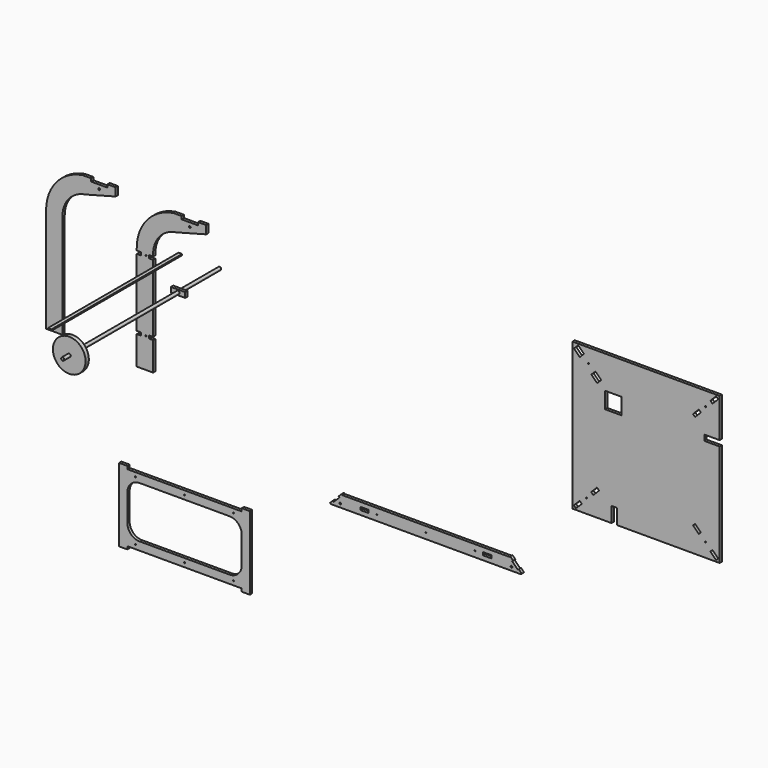
from build123d import *

# Parameters (mm, degrees)
F0_R          = 3.302
F0_R_2        = 5.588
F1_DEPTH      = 18.034
F0_W          = 50.8
F0_H          = 18.034
F0_W_2        = 101.6
F0_H_2        = 101.6
F0_W_3        = 88.9
F0_H_3        = 31.75
F0_R_3        = 9.525
F0_W_4        = 22.225
F0_H_4        = 7.62
F2_DEPTH      = 1016
F3_DEPTH      = 914.4
F3_DEPTH_BACK = 304.8
F5_START      = -50.8
F4_R          = 101.6
F4_R_2        = 9.525
F5_DEPTH      = 25.4


# Not quite as in the source:
# - a feature names something its author has since deleted; it is built from what else it names


with BuildPart() as f1:
    # F0 (on Front) → F1 (new body)
    with BuildSketch(Plane.XZ):
        with BuildLine():
            Line((-256.7524378796, -311.5848713337), (-256.7524378796, -489.3848713337))
            Line((-256.7524378796, -489.3848713337), (-155.1524378796, -489.3848713337))
            Line((-155.1524378796, -489.3848713337), (-155.1524378796, -311.5848713337))
            Line((-155.1524378796, -311.5848713337), (-180.5524378796, -311.5848713337))
            Line((-180.5524378796, -311.5848713337), (-180.5524378796, -293.5508713337))
            Line((-180.5524378796, -293.5508713337), (-155.1524378796, -293.5508713337))
            Line((-155.1524378796, -293.5508713337), (-155.1524378796, 127.5811286663))
            Line((-155.1524378796, 127.5811286663), (-180.5524378796, 127.5811286663))
            Line((-180.5524378796, 127.5811286663), (-180.5524378796, 145.6151286663))
            Line((-180.5524378796, 145.6151286663), (-155.1524378796, 145.6151286663))
            Line((-155.1524378796, 145.6151286663), (-155.1524378796, 159.8593657013))
            ThreePointArc((-155.1524378796, 159.8593657013), (-114.7622837077, 268.5646027694), (-13.1903100775, 324.5228666178))
            Line((-13.1903100775, 324.5228666178), (175.0475621204, 374.6868958044))
            Line((175.0475621204, 374.6868958044), (175.0475621204, 406.9811286663))
            Line((175.0475621204, 406.9811286663), (175.0475621204, 425.0151286663))
            Line((175.0475621204, 425.0151286663), (124.2475621204, 425.0151286663))
            Line((124.2475621204, 425.0151286663), (124.2475621204, 406.9811286663))
            Line((124.2475621204, 406.9811286663), (22.6475621204, 406.9811286663))
            Line((22.6475621204, 406.9811286663), (22.6475621204, 425.0151286663))
            Line((22.6475621204, 425.0151286663), (-28.1524378796, 425.0151286663))
            ThreePointArc((-28.1524378796, 425.0151286663), (-191.7126319353, 334.9061727512), (-256.7524378796, 159.8593657013))
            Line((-256.7524378796, 159.8593657013), (-256.7524378796, 145.6151286663))
            Line((-256.7524378796, 145.6151286663), (-231.3524378796, 145.6151286663))
            Line((-231.3524378796, 145.6151286663), (-231.3524378796, 127.5811286663))
            Line((-231.3524378796, 127.5811286663), (-256.7524378796, 127.5811286663))
            Line((-256.7524378796, 127.5811286663), (-256.7524378796, -293.5508713337))
            Line((-256.7524378796, -293.5508713337), (-231.3524378796, -293.5508713337))
            Line((-231.3524378796, -293.5508713337), (-231.3524378796, -311.5848713337))
            Line((-231.3524378796, -311.5848713337), (-256.7524378796, -311.5848713337))
        make_face()
        with Locations((-199.6024378796, -302.5678713337)):
            Circle(F0_R, mode=Mode.SUBTRACT)
        with Locations((-199.6024378796, 136.5981286663)):
            Circle(F0_R, mode=Mode.SUBTRACT)
        with Locations((73.4475621204, 381.5811286663)):
            Circle(F0_R_2, mode=Mode.SUBTRACT)
    extrude(amount=F1_DEPTH)


with BuildPart() as f1b:
    # F0 (on Front) → F1, piece 2 (new body)
    with BuildSketch(Plane.XZ):
        with BuildLine():
            ThreePointArc((-718.6880954381, 183.6058530265), (-678.2979412662, 292.3110900946), (-576.7259676359, 348.269353943))
            Line((-576.7259676359, 348.269353943), (-388.488095438, 398.4333831296))
            Line((-388.4880954381, 398.4333831296), (-388.4880954381, 430.7276159915))
            Line((-388.4880954381, 430.7276159915), (-388.4880954381, 448.7616159915))
            Line((-388.4880954381, 448.7616159915), (-439.2880954381, 448.7616159915))
            Line((-439.2880954381, 448.7616159915), (-439.2880954381, 430.7276159915))
            Line((-439.2880954381, 430.7276159915), (-540.8880954381, 430.7276159915))
            Line((-540.8880954381, 430.7276159915), (-540.8880954381, 448.7616159915))
            Line((-540.8880954381, 448.7616159915), (-591.6880954381, 448.7616159915))
            ThreePointArc((-591.6880954381, 448.7616159915), (-755.2482894938, 358.6526600765), (-820.2880954381, 183.6058530265))
            Line((-820.2880954381, 183.6058530265), (-820.2880954381, -465.6383840085))
            Line((-820.2880954381, -465.6383840085), (-718.6880954381, -465.6383840085))
            Line((-718.6880954381, -465.6383840085), (-718.6880954381, 183.6058530265))
        make_face()
        with Locations((-490.0880954381, 405.3276159915)):
            Circle(F0_R_2, mode=Mode.SUBTRACT)
    extrude(amount=F1_DEPTH)


with BuildPart() as f1c:
    # F0 (on Front) → F1, piece 3 (new body)
    with BuildSketch(Plane.XZ):
        Polygon((-315.3730721781, -1069.7679861069), (-366.1730721781, -1069.7679861069), (-366.1730721781, -1490.8999861069), (-315.3730721781, -1490.8999861069), (395.8269278219, -1490.8999861069), (446.6269278219, -1490.8999861069), (446.6269278219, -1069.7679861069), (395.8269278219, -1069.7679861069), align=None)
        with Locations((-264.5730721781, -1465.4999861069)):
            Circle(F0_R, mode=Mode.SUBTRACT)
        with Locations((40.2269278219, -1465.4999861069)):
            Circle(F0_R, mode=Mode.SUBTRACT)
        with BuildLine():
            ThreePointArc((-315.3730721781, -1196.7679861069), (-293.0546089045, -1142.8864493805), (-239.1730721781, -1120.5679861069))
            Line((-239.1730721781, -1120.5679861069), (319.6269278219, -1120.5679861069))
            ThreePointArc((319.6269278219, -1120.5679861069), (373.5084645483, -1142.8864493805), (395.8269278219, -1196.7679861069))
            Line((395.8269278219, -1196.7679861069), (395.8269278219, -1363.8999861069))
            ThreePointArc((395.8269278219, -1363.8999861069), (373.5084645483, -1417.7815228333), (319.6269278219, -1440.0999861069))
            Line((319.6269278219, -1440.0999861069), (-239.1730721781, -1440.0999861069))
            ThreePointArc((-239.1730721781, -1440.0999861069), (-293.0546089045, -1417.7815228333), (-315.3730721781, -1363.8999861069))
            Line((-315.3730721781, -1363.8999861069), (-315.3730721781, -1196.7679861069))
        make_face(mode=Mode.SUBTRACT)
        with Locations((-264.5730721781, -1095.1679861069)):
            Circle(F0_R, mode=Mode.SUBTRACT)
        with Locations((40.2269278219, -1095.1679861069)):
            Circle(F0_R, mode=Mode.SUBTRACT)
        with Locations((345.0269278219, -1465.4999861069)):
            Circle(F0_R, mode=Mode.SUBTRACT)
        with Locations((345.0269278219, -1095.1679861069)):
            Circle(F0_R, mode=Mode.SUBTRACT)
        with Locations((-340.7730721781, -1060.7509861069)):
            Rectangle(F0_W, F0_H)
        with Locations((421.2269278219, -1060.7509861069)):
            Rectangle(F0_W, F0_H)
        with Locations((421.2269278219, -1499.9169861069)):
            Rectangle(F0_W, F0_H)
        with Locations((-340.7730721781, -1499.9169861069)):
            Rectangle(F0_W, F0_H)
    extrude(amount=F1_DEPTH)


with BuildPart() as f1d:
    # F0 (on Front) → F1, piece 4 (new body)
    with BuildSketch(Plane.XZ):
        Polygon((2728.8376075736, -291.5323071868), (2728.8376075736, -385.9785684254), (3365.8825668832, -385.9785684254), (3365.8825668832, 251.3926928132), (3270.6325668832, 251.3926928132), (3270.6325668832, 286.3176928132), (3365.8825668832, 286.3176928132), (3365.8825668832, 528.4214315746), (2451.4825668832, 528.4214315746), (2451.4825668832, -385.9785684254), (2693.9126075736, -385.9785684254), (2693.9126075736, -291.5323071868), align=None)
        Polygon((2496.0684305155, -328.6407411012), (2508.8203942074, -341.3927047931), (2472.8993697231, -377.3137292774), (2460.1474060312, -364.5617655855), align=None, mode=Mode.SUBTRACT)
        with Locations((2538.3654368457, -299.0956984629)):
            Circle(F0_R, mode=Mode.SUBTRACT)
        Polygon((2603.8315039683, -220.8776676484), (2616.5834676602, -233.6296313403), (2580.662443176, -269.5506558246), (2567.910479484, -256.7986921326), align=None, mode=Mode.SUBTRACT)
        Polygon((3357.2177277351, -364.5617655855), (3344.4657640432, -377.3137292774), (3308.5447395589, -341.3927047931), (3321.2967032509, -328.6407411012), align=None, mode=Mode.SUBTRACT)
        Polygon((3249.4546542823, -256.7986921326), (3236.7026905904, -269.5506558246), (3200.7816661061, -233.6296313403), (3213.533629798, -220.8776676484), align=None, mode=Mode.SUBTRACT)
        with Locations((3278.9996969206, -299.0956984629)):
            Circle(F0_R, mode=Mode.SUBTRACT)
        with Locations((2705.4825668832, 274.4214315746)):
            Rectangle(F0_W_2, F0_H_2, mode=Mode.SUBTRACT)
        Polygon((2568.7111476991, 386.3110991977), (2594.2493832335, 411.7806722172), (2630.1704077178, 375.8596477329), (2604.6664803341, 350.3557203489), align=None, mode=Mode.SUBTRACT)
        with Locations((2551.796844501, 441.1701824532)):
            Circle(F0_R, mode=Mode.SUBTRACT)
        Polygon((2486.4863097807, 519.5437456699), (2522.407334265, 483.6227211856), (2496.9377612456, 458.0844856513), (2460.9823823967, 494.0398182862), align=None, mode=Mode.SUBTRACT)
        Polygon((3200.7816661061, 376.0724944895), (3236.7026905904, 411.9935189737), (3249.4546542823, 399.2415552818), (3213.533629798, 363.3205307975), align=None, mode=Mode.SUBTRACT)
        with Locations((3278.9996969206, 441.538561612)):
            Circle(F0_R, mode=Mode.SUBTRACT)
        Polygon((3321.2967032509, 471.0836042504), (3308.5447395589, 483.8355679423), (3344.4657640432, 519.7565924266), (3357.2177277351, 507.0046287346), align=None, mode=Mode.SUBTRACT)
    extrude(amount=F1_DEPTH)


with BuildPart() as f1e:
    # F0 (on Front) → F1, piece 5 (new body)
    with BuildSketch(Plane.XZ):
        Polygon((967.6722639506, -831.2486945482), (949.7117517085, -849.2092067904), (2130.8015917085, -849.2092067904), (2112.8410794663, -831.2486945482), (2076.9200549821, -795.3276700639), (2058.9595427399, -777.3671578218), (1021.553800677, -777.3671578218), (1003.5932884349, -795.3276700639), align=None)
        with Locations((1008.0834164954, -826.7585664877)):
            Circle(F0_R_2, mode=Mode.SUBTRACT)
        with Locations((1159.2566717085, -813.2881823061)):
            Rectangle(F0_W, F0_H, mode=Mode.SUBTRACT)
        with Locations((1235.4566717085, -813.2881823061)):
            Circle(F0_R, mode=Mode.SUBTRACT)
        with Locations((1540.2566717085, -813.2881823061)):
            Circle(F0_R, mode=Mode.SUBTRACT)
        with Locations((1845.0566717085, -813.2881823061)):
            Circle(F0_R, mode=Mode.SUBTRACT)
        with Locations((1921.2566717085, -813.2881823061)):
            Rectangle(F0_W, F0_H, mode=Mode.SUBTRACT)
        with Locations((2072.4299269215, -826.7585664877)):
            Circle(F0_R_2, mode=Mode.SUBTRACT)
        Polygon((944.6828082807, -844.1802633626), (949.7117517085, -849.2092067904), (967.6722639506, -831.2486945482), (962.6433205228, -826.2197511204), align=None)
        Polygon((998.5643450071, -790.2987266361), (1003.5932884349, -795.3276700639), (1021.553800677, -777.3671578218), (1016.5248572492, -772.338214394), align=None)
        Polygon((2058.9595427399, -777.3671578218), (2076.9200549821, -795.3276700639), (2081.9489984099, -790.2987266361), (2063.9884861677, -772.338214394), align=None)
        Polygon((2112.8410794663, -831.2486945482), (2130.8015917085, -849.2092067904), (2135.8305351363, -844.1802633626), (2117.8700228941, -826.2197511204), align=None)
    extrude(amount=F1_DEPTH)


with BuildPart() as f1f:
    # F0 (on Front) → F1, piece 6 (new body)
    with BuildSketch(Plane.XZ):
        Rectangle(F0_W_3, F0_H_3)
        Circle(F0_R_3, mode=Mode.SUBTRACT)
    extrude(amount=F1_DEPTH)

    # F0 (on Front) → F3 (join, two sides)
    with BuildSketch(Plane.XZ) as f3_sk:
        Circle(F0_R_3)
    extrude(amount=F3_DEPTH)
    extrude(f3_sk.sketch, amount=-F3_DEPTH_BACK)

    # F4 (on face) → F5 (join)
    with BuildSketch(Plane.XZ.offset(914.4).offset(F5_START)):
        Circle(F4_R)
        Circle(F4_R_2, mode=Mode.SUBTRACT)
    extrude(amount=-F5_DEPTH)


with BuildPart() as f2:
    # F0 (on Front) → F2 (new body)
    with BuildSketch(Plane.XZ):
        with Locations((0, 203.2)):
            Rectangle(F0_W_4, F0_H_4)
    extrude(amount=F2_DEPTH)


solid = Compound([f1.part, f1b.part, f1c.part, f1d.part, f1e.part, f1f.part, f2.part])
